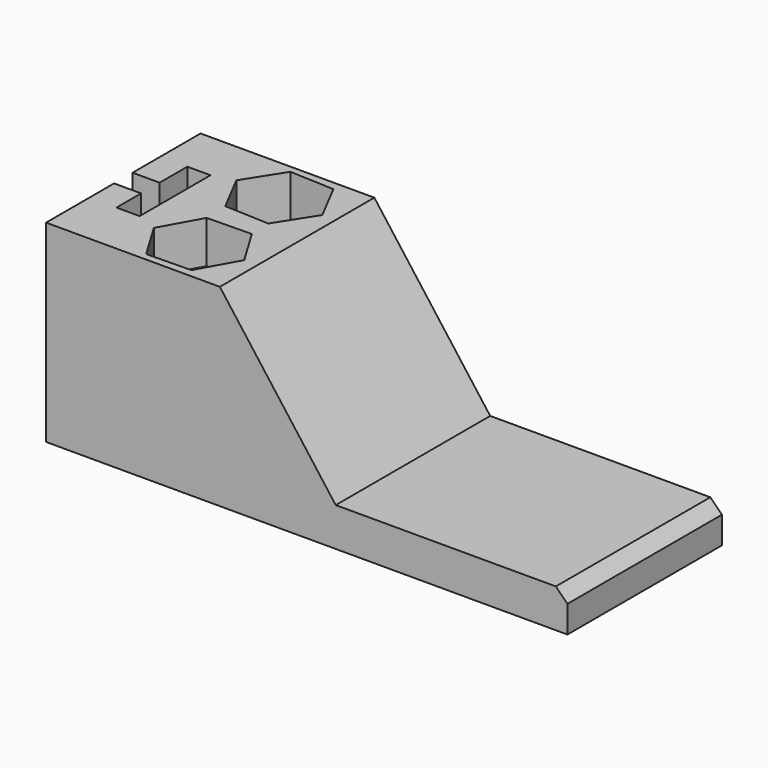
from build123d import *

# Parameters (mm, degrees)
F1_DEPTH       = 25
F2_DEPTH       = 25
F4_D           = 13.2
F4_CBORE_D     = 23
F4_CBORE_DEPTH = 0
F6_DEPTH       = 50.001
F8_DEPTH       = 11
F9_SIZE        = 3


# Not quite as in the source:
# - a feature names something its author has since deleted; it is built from what else it names


with BuildPart() as f1:
    # F0 (on Front) → F1 (new body, symmetric)
    with BuildSketch(Plane.XZ):
        Polygon((67.5, -5), (67.5, 5), (7.5, 5), (-67.5, 5), (-67.5, -5), align=None)
    extrude(amount=F1_DEPTH, both=True)

    # F0 (on Front) → F2 (join, symmetric)
    with BuildSketch(Plane.XZ):
        Polygon((-67.5, 5), (7.5, 5), (-22.5, 45), (-67.5, 45), align=None)
    extrude(amount=F2_DEPTH, both=True)

    # F4 (through all)
    with Locations(Plane(origin=(0, 0, -5), x_dir=(1, 0, 0), z_dir=(0, 0, -1))):
        with Locations((-37.5, 13), (-37.5, -13)):
            CounterBoreHole(F4_D / 2, F4_CBORE_D / 2, F4_CBORE_DEPTH)

    # F5 (on face) → F6 (cut, through all)
    with BuildSketch(Plane.XY.offset(45)):
        Polygon((-60.5, 3), (-67.5, 3), (-67.5, -3), (-60.5, -3), (-60.5, -10.9647801146), (-54.5, -10.9647801146), (-54.5, 11.965367943), (-60.5, 11.965367943), align=None)
    extrude(amount=-F6_DEPTH, mode=Mode.SUBTRACT)

    # F7 (on face) → F8 (cut)
    with BuildSketch(Plane.XY.offset(45)):
        Polygon((-25.954678559, -12.8028042668), (-31.898115794, -2.9028604706), (-43.443437235, -3.1000562039), (-49.045321441, -13.1971957332), (-43.101884206, -23.0971395294), (-31.556562765, -22.8999437961), align=None)
        Polygon((-25.9640170016, 12.4955898546), (-31.2951765009, 22.7382492615), (-42.8311594993, 23.2426594069), (-49.0359829984, 13.5044101454), (-43.7048234991, 3.2617507385), (-32.1688405007, 2.7573405931), align=None)
    extrude(amount=-F8_DEPTH, mode=Mode.SUBTRACT)

    # F9
    f9_edges = [f1.edges().sort_by_distance(p)[0] for p in [
        (67.5, 0, 5),
    ]]
    chamfer(f9_edges, length=F9_SIZE)


solid = f1.part
